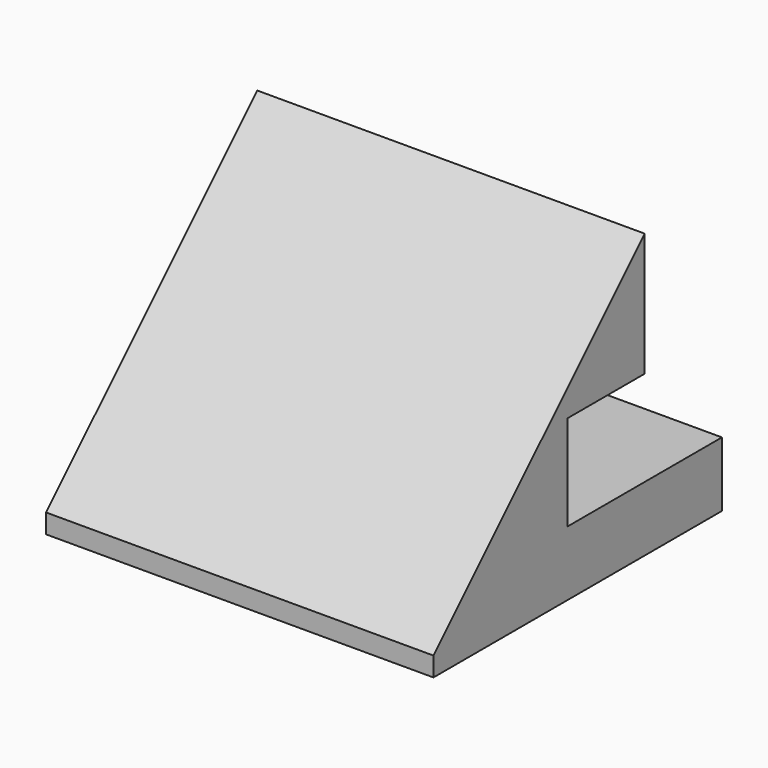
from build123d import *

# Parameters (mm, degrees)
F0_W        = 100.3427430987
F0_H        = 68.4072636068
F1_DEPTH    = 75
F2_T1_DEPTH = 460.378361414
F3_W        = 100.3427430987
F3_H        = 24.6774237603
F4_DEPTH    = 25
F5_DEPTH    = 25


# Not quite as in the source:
# - a fillet or chamfer that OpenCascade refuses, or shapes differently, is made with other operations: its cross-section is extruded or revolved along the edge and cut away or added


with BuildPart() as f1:
    # F0 (on Top) → F1 (new body)
    with BuildSketch(Plane.XY):
        with Locations((-2.3588724434, -1.9959677011)):
            Rectangle(F0_W, F0_H)
    extrude(amount=F1_DEPTH)

    # F2: chamfer of 70 on 1 edges, made by hand

    # F2_s2 → F2_t1 (cut)
    with BuildSketch(Plane.YZ.offset(-232.5480531504)):
        Polygon((-36.1995995045, 5), (33.8004004955, 75), (-36.1995995045, 75), align=None)
    extrude(amount=F2_T1_DEPTH, mode=Mode.SUBTRACT)

    # F3 (on face) → F4 (cut)
    with BuildSketch(Plane(origin=(0, 32.2076641023, 0), x_dir=(-1, 0, 0), z_dir=(0, 1, 0))):
        with Locations((2.3588724434, 29.1229868308)):
            Rectangle(F3_W, F3_H)
    extrude(amount=-F4_DEPTH, mode=Mode.SUBTRACT)

    # F5 (add): a face of the model
    f5_faces = [f1.faces().sort_by_distance(p)[0] for p in [
        (-2.3588724434, 32.2076641023, 8.3921374753),
    ]]
    extrude(f5_faces, amount=F5_DEPTH)


solid = f1.part
